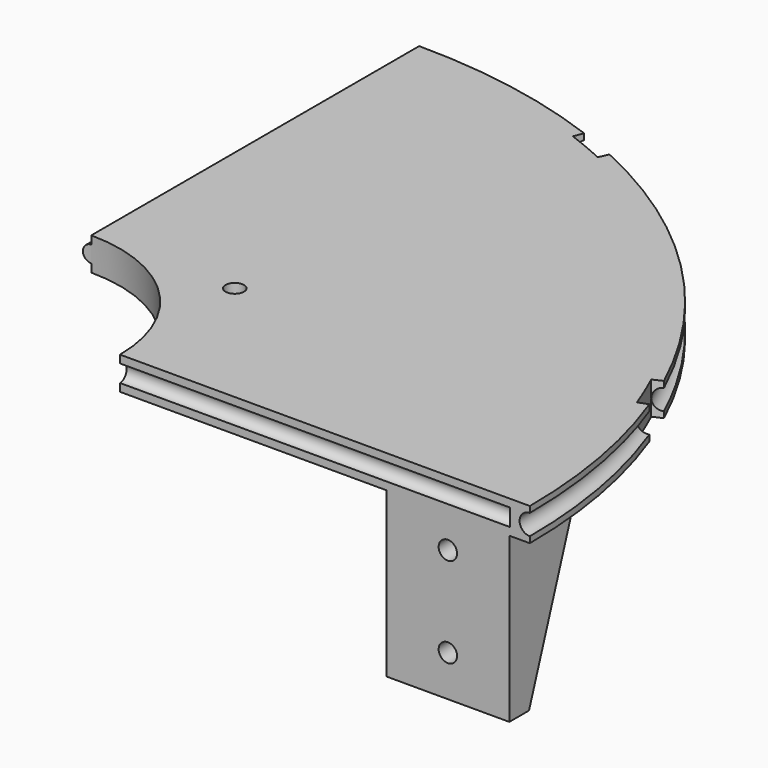
from build123d import *

# Parameters (mm, degrees)
F0_R         = 2.25
F1_DEPTH     = 8
F4_R         = 2.5
F6_W         = 30
F6_H         = 20
F6_W_2       = 20
F6_H_2       = 30
F7_DEPTH     = 40
F8_W         = 15
F8_H         = 14
F8_W_2       = 14
F8_H_2       = 15
F9_DEPTH     = 40
F10_SIZE2    = 39.99999
F10_SIZE     = 13.99999
F10_2_SIZE2  = 39.99999
F10_2_SIZE   = 13.99999
F11_R        = 2.25
F12_DEPTH    = 25
F14_R        = 2.25
F15_DEPTH    = 25
F17_DEPTH    = 25
F20_R        = 2
F23_DEPTH    = 48.001
F24_R        = 2.1
F27_DEPTH    = 4
F28_T1_DEPTH = 4


# Not quite as in the source:
# - a fillet or chamfer that OpenCascade refuses, or shapes differently, is made with other operations: its cross-section is extruded or revolved along the edge and cut away or added
# - two fillets or chamfers of one size are made in one step
# - a fillet or chamfer is up to 0.001 mm smaller than in the source, because OpenCascade refuses the exact size


with BuildPart() as f1:
    # F0 (on Top) → F1 (new body)
    with BuildSketch(Plane.XY):
        with BuildLine():
            Line((35, 0), (135, 0))
            ThreePointArc((135, 0), (95.4594154602, 95.4594154602), (0, 135))
            Line((0, 135), (0, 35))
            ThreePointArc((0, 35), (24.7487373415, 24.7487373415), (35, 0))
        make_face()
        with Locations((35, 35)):
            Circle(F0_R, mode=Mode.SUBTRACT)
    extrude(amount=F1_DEPTH)

    # F5: sweep along a path in F3
    with BuildLine(Plane.XY.offset(4)) as f5_path:
        CenterArc((0, 0), 135, 0, 360)
    # F4 (on face) → F5 (sweep, cut)
    with BuildSketch(Plane.XZ):
        with Locations((135, 4)):
            Circle(F4_R)
    sweep(path=f5_path.line, mode=Mode.SUBTRACT)

    # F6 (on face) → F7 (join)
    with BuildSketch(Plane(origin=(0, 0, 0), x_dir=(1, 0, 0), z_dir=(0, 0, -1))):
        with Locations((115, -10)):
            Rectangle(F6_W, F6_H)
        with Locations((10, -115)):
            Rectangle(F6_W_2, F6_H_2)
    extrude(amount=F7_DEPTH)

    # F8 (on face) → F9 (cut)
    with BuildSketch(Plane(origin=(0, 0, -40), x_dir=(1, 0, 0), z_dir=(0, 0, -1))):
        with Locations((115, -13)):
            Rectangle(F8_W, F8_H)
        with Locations((13, -115)):
            Rectangle(F8_W_2, F8_H_2)
    extrude(amount=-F9_DEPTH, mode=Mode.SUBTRACT)

    # F10 (size 14 and 40 in the source; OpenCascade refuses exactly that, so slightly less here)
    f10_edges = [f1.edges().sort_by_distance(p)[0] for p in [
        (103.75, 20, -40),
        (126.25, 20, -40),
    ]]
    f10_side = f1.faces().sort_by_distance((129.639445, 10, -40))[0]
    chamfer(f10_edges, length=F10_SIZE, length2=F10_SIZE2, reference=f10_side)

    # F10#2 (size 14 and 40 in the source; OpenCascade refuses exactly that, so slightly less here)
    f10_2_edges = [f1.edges().sort_by_distance(p)[0] for p in [
        (20, 103.75, -40),
        (20, 126.25, -40),
    ]]
    f10_2_side = f1.faces().sort_by_distance((19.639445, 103.75, -40))[0]
    chamfer(f10_2_edges, length=F10_2_SIZE, length2=F10_2_SIZE2, reference=f10_2_side)

    # F11 (on face) → F12 (cut)
    with BuildSketch(Plane(origin=(0, 6, 0), x_dir=(-1, 0, 0), z_dir=(0, 1, 0))):
        with Locations((-115, -8)):
            Circle(F11_R)
        with Locations((-115, -30)):
            Circle(F11_R)
    extrude(amount=-F12_DEPTH, mode=Mode.SUBTRACT)

    # F14 (on face) → F15 (cut)
    with BuildSketch(Plane.YZ.offset(6)):
        with Locations((115, -30)):
            Circle(F14_R)
        with Locations((115, -8)):
            Circle(F14_R)
    extrude(amount=-F15_DEPTH, mode=Mode.SUBTRACT)

    # F16 (on face) → F17 (cut)
    with BuildSketch(Plane.XY.offset(8)):
        with BuildLine():
            ThreePointArc((120.4496071259, 55.2099822787), (122.4117800348, 50.7110057948), (124.2059779255, 46.1424430169))
            Line((124.2059779255, 46.1424430169), (126.549486943, 47.0130551493))
            ThreePointArc((126.549486943, 47.0130551493), (124.7214362618, 51.6678172249), (122.7222412226, 56.2516800575))
            Line((122.7222412226, 56.2516800575), (120.4496071259, 55.2099822787))
        make_face()
        with BuildLine():
            Line((47.0017845491, 126.5536733928), (46.1313811315, 124.2100868484))
            ThreePointArc((46.1313811315, 124.2100868484), (50.7001036814, 122.416295838), (55.1992548973, 120.4545236128))
            Line((55.1992548973, 120.4545236128), (56.2407502727, 122.7272504734))
            ThreePointArc((56.2407502727, 122.7272504734), (51.6567094112, 124.7260372689), (47.0017845491, 126.5536733928))
        make_face()
    extrude(amount=-F17_DEPTH, mode=Mode.SUBTRACT)

    # F21: sweep along a path in F19
    with BuildLine(Plane(origin=(0, 0, 0), x_dir=(0, -1, 0), z_dir=(-1, 0, 0))) as f21_path:
        Line((-130, 4), (0, 4))
    # F20 (on Front) → F21 (sweep)
    with BuildSketch(Plane.XZ):
        with Locations((0, 4)):
            Circle(F20_R)
    sweep(path=f21_path.line)

    # F22 (on face) → F23 (cut, through all)
    with BuildSketch(Plane.XY.offset(8)):
        with BuildLine():
            ThreePointArc((0, 35), (-24.7487373415, -24.7487373415), (35, 0))
            ThreePointArc((35, 0), (24.7487373415, 24.7487373415), (0, 35))
        make_face()
    extrude(amount=-F23_DEPTH, mode=Mode.SUBTRACT)

    # F25: sweep along a path in F18
    with BuildLine(Plane.XZ) as f25_path:
        Line((0, 4), (130.2, 4))
    # F24 (on Right) → F25 (sweep, cut)
    with BuildSketch(Plane.YZ):
        with Locations((0, 4)):
            Circle(F24_R)
    sweep(path=f25_path.line, mode=Mode.SUBTRACT)

    # F26 (on face) → F27 (cut)
    with BuildSketch(Plane(origin=(0, 0, 0), x_dir=(1, 0, 0), z_dir=(0, 0, -1))):
        with BuildLine():
            Line((37, -40), (13, -40))
            ThreePointArc((13, -40), (9.4644660941, -41.4644660941), (8, -45))
            Line((8, -45), (8, -100))
            Line((8, -100), (20, -100))
            Line((20, -100), (20, -122.5))
            ThreePointArc((20, -122.5), (87.7674484077, -87.7674484077), (122.5, -20))
            Line((122.5, -20), (100, -20))
            Line((100, -20), (100, -8))
            Line((100, -8), (45, -8))
            ThreePointArc((45, -8), (41.4644660941, -9.4644660941), (40, -13))
            Line((40, -13), (40, -37))
            ThreePointArc((40, -37), (39.1213203436, -39.1213203436), (37, -40))
        make_face()
    extrude(amount=-F27_DEPTH, mode=Mode.SUBTRACT)

    # F28: fillet of radius 5 on 4 edges, made by hand

    # F28_s2 → F28_t1 (join)
    with BuildSketch(Plane.XY):
        with BuildLine():
            ThreePointArc((100, 13), (98.5355339059, 9.4644660941), (95, 8))
            Line((95, 8), (100, 8))
            Line((100, 8), (100, 13))
        make_face()
        with BuildLine():
            ThreePointArc((13, 100), (9.4644660941, 98.5355339059), (8, 95))
            Line((8, 95), (8, 100))
            Line((8, 100), (13, 100))
        make_face()
        with BuildLine():
            ThreePointArc((26.0493451107, 121.3576599119), (21.8572882373, 120.3578891664), (20, 116.469012365))
            Line((20, 116.469012365), (20, 122.5))
            ThreePointArc((20, 122.5), (23.0317559361, 121.9663405145), (26.0493451107, 121.3576599119))
        make_face()
        with BuildLine():
            ThreePointArc((121.3576599119, 26.0493451107), (120.3578891664, 21.8572882373), (116.469012365, 20))
            Line((116.469012365, 20), (122.5, 20))
            ThreePointArc((122.5, 20), (121.9663405145, 23.0317559361), (121.3576599119, 26.0493451107))
        make_face()
    extrude(amount=F28_T1_DEPTH)


solid = f1.part
